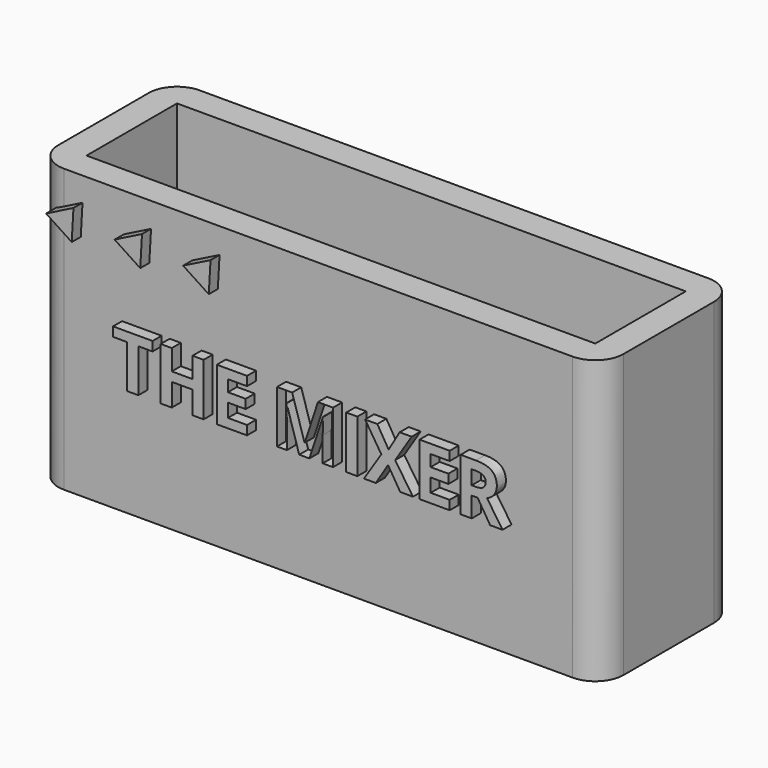
from build123d import *

# Parameters (mm, degrees)
F0_W         = 100
F0_H         = 30
F1_DEPTH     = 50
F2_T         = -5
F3_TEXT_SIZE = 12.987012987
F4_DEPTH     = 2
F5_T1_DEPTH  = 75
F5_T6_DEPTH  = 75
F5_T12_DEPTH = 75
F5_T18_DEPTH = 75
F7_D         = 20
F7_DEPTH     = 12
F7_TIP       = 6.0086061903


# Not quite as in the source:
# - a fillet or chamfer that OpenCascade refuses, or shapes differently, is made with other operations: its cross-section is extruded or revolved along the edge and cut away or added
# - Text() gives the source's letters only with a copy of the font that has no kerning and outlines rounded to 1/6400 em; it was checked with that copy


with BuildPart() as f1:
    # F0 (on Top) → F1 (new body)
    with BuildSketch(Plane.XY):
        with Locations((3.9354469627, -9.713625235)):
            Rectangle(F0_W, F0_H)
    extrude(amount=F1_DEPTH)

    # F2
    f2_openings = [f1.faces().sort_by_distance(p)[0] for p in [
        (3.935447, -9.713625, 50),
    ]]
    offset(amount=F2_T, openings=f2_openings)

    # F3 (on face) → F4 (join)
    with BuildSketch(Plane.XZ.offset(24.713625235)):
        Polygon((-38.0868242341, 40.342835477), (-37.7778671682, 45.7584634423), (-42.6224170965, 43.3182141274), align=None)
        Polygon((-25.9644071375, 40.2246213496), (-25.6554500716, 45.6402493149), (-30.5, 43.2), align=None)
        Polygon((-13.841990041, 40.1064072222), (-13.5330329751, 45.5220351875), (-18.3775829035, 43.0817858726), align=None)
        with Locations((-31.0426133292, 20.3246753247)):
            Text('THE MIXER', F3_TEXT_SIZE, font='Open Sans', font_style=FontStyle.BOLD, text_align=(TextAlign.LEFT, TextAlign.BOTTOM))
    extrude(amount=F4_DEPTH)

    # F5: fillet of radius 5 on 4 edges, made by hand

    # F5_s2 → F5_t1 (cut)
    with BuildSketch(Plane.XY.offset(-12.5)):
        with BuildLine():
            ThreePointArc((53.9354469627, -19.713625235), (52.4709808686, -23.249159141), (48.9354469627, -24.713625235))
            Line((48.9354469627, -24.713625235), (53.9354469627, -24.713625235))
            Line((53.9354469627, -24.713625235), (53.9354469627, -19.713625235))
        make_face()
        with BuildLine():
            ThreePointArc((48.9354469627, 5.286374765), (52.4709808686, 3.8219086709), (53.9354469627, 0.286374765))
            Line((53.9354469627, 0.286374765), (53.9354469627, 5.286374765))
            Line((53.9354469627, 5.286374765), (48.9354469627, 5.286374765))
        make_face()
        with BuildLine():
            ThreePointArc((-41.0645530373, 5.286374765), (-44.6000869432, 3.8219086709), (-46.0645530373, 0.286374765))
            Line((-46.0645530373, 0.286374765), (-46.0645530373, 5.286374765))
            Line((-46.0645530373, 5.286374765), (-41.0645530373, 5.286374765))
        make_face()
    extrude(amount=F5_T1_DEPTH, mode=Mode.SUBTRACT)


with BuildPart() as f5_tool4:
    # F5_s5 → F5_t6 (new body)
    with BuildSketch(Plane.XY.offset(-12.5)):
        with BuildLine():
            ThreePointArc((-46.0645530373, -19.713625235), (-44.6000869432, -23.249159141), (-41.0645530373, -24.713625235))
            Line((-41.0645530373, -24.713625235), (-46.0645530373, -24.713625235))
            Line((-46.0645530373, -24.713625235), (-46.0645530373, -19.713625235))
        make_face()
    extrude(amount=F5_T6_DEPTH)

    split(bisect_by=Plane(origin=(7.0435511577, 0, 10.7370133724), x_dir=(0, 1, 0), z_dir=(-0.5485141541, 0, -0.8361412696)), keep=Keep.TOP)

    split(bisect_by=Plane(origin=(-26.029777802, 0, 51.6760961329), x_dir=(0, 1, 0), z_dir=(0.4498625036, 0, -0.8930978266)), keep=Keep.TOP)


with BuildPart() as f1_1:
    add(f1.part)

    # F5_t3: cut F5_tool4
    add(f5_tool4.part, mode=Mode.SUBTRACT)


with BuildPart() as f5_tool10:
    # F5_s11 → F5_t12 (new body)
    with BuildSketch(Plane.XY.offset(-12.5)):
        with BuildLine():
            ThreePointArc((-46.0645530373, -19.713625235), (-44.6000869432, -23.249159141), (-41.0645530373, -24.713625235))
            Line((-41.0645530373, -24.713625235), (-46.0645530373, -24.713625235))
            Line((-46.0645530373, -24.713625235), (-46.0645530373, -19.713625235))
        make_face()
    extrude(amount=F5_T12_DEPTH)

    split(bisect_by=Plane(origin=(7.0435511577, 0, 10.7370133724), x_dir=(0, 1, 0), z_dir=(-0.5485141541, 0, -0.8361412696)), keep=Keep.TOP)

    split(bisect_by=Plane(origin=(-26.029777802, 0, 51.6760961329), x_dir=(0, 1, 0), z_dir=(-0.4498625036, 0, 0.8930978266)), keep=Keep.TOP)


with BuildPart() as f1_2:
    add(f1_1.part)

    # F5_t9: cut F5_tool10
    add(f5_tool10.part, mode=Mode.SUBTRACT)


with BuildPart() as f5_tool16:
    # F5_s17 → F5_t18 (new body)
    with BuildSketch(Plane.XY.offset(-12.5)):
        with BuildLine():
            ThreePointArc((-46.0645530373, -19.713625235), (-44.6000869432, -23.249159141), (-41.0645530373, -24.713625235))
            Line((-41.0645530373, -24.713625235), (-46.0645530373, -24.713625235))
            Line((-46.0645530373, -24.713625235), (-46.0645530373, -19.713625235))
        make_face()
    extrude(amount=F5_T18_DEPTH)

    split(bisect_by=Plane(origin=(7.0435511577, 0, 10.7370133724), x_dir=(0, 1, 0), z_dir=(0.5485141541, 0, 0.8361412696)), keep=Keep.TOP)

    split(bisect_by=Plane(origin=(-26.029777802, 0, 51.6760961329), x_dir=(0, 1, 0), z_dir=(-0.4498625036, 0, 0.8930978266)), keep=Keep.TOP)


with BuildPart() as f1_3:
    add(f1_2.part)

    # F5_t15: cut F5_tool16
    add(f5_tool16.part, mode=Mode.SUBTRACT)

    # F7
    with Locations(Plane(origin=(0, 5.286374765, 0), x_dir=(-1, 0, 0), z_dir=(0, 1, 0))):
        with Locations((-3.9350690715, 25.0547545797)):
            Hole(F7_D / 2, depth=F7_DEPTH)
            with Locations((0, 0, -(F7_DEPTH + F7_TIP / 2))):  # 118° drill point
                Cone(0, F7_D / 2, F7_TIP, mode=Mode.SUBTRACT)


solid = f1_3.part
